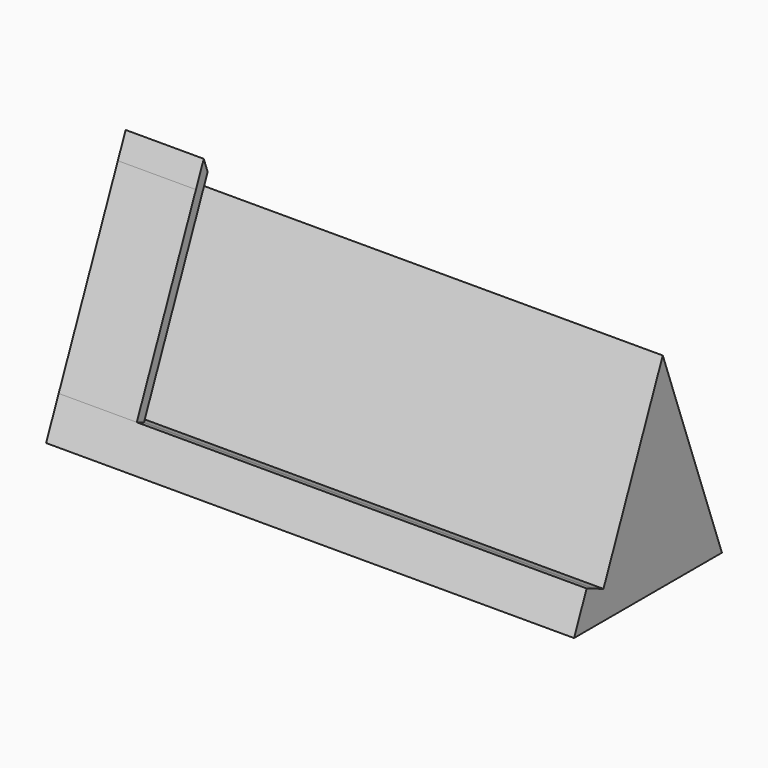
from build123d import *

# Parameters (mm, degrees)
F1_DEPTH = 57.6
F2_DEPTH = 5
F3_START = -5
F3_DEPTH = 5


# Not quite as in the source:
# - a feature names something its author has since deleted; it is built from what else it names


with BuildPart() as f1:
    # F0 (on Right) → F1 (new body)
    with BuildSketch(Plane.YZ):
        Polygon((1.5365748771, 3.633035603), (0, 0), (20.4984284937, 0), (11.0311029763, 26.0816380962), align=None)
        Polygon((0, 4.2829225325), (0, 0), (1.5365748771, 3.633035603), align=None)
        Polygon((-1.811441418, 0), (0, 0), (0, 4.2829225325), align=None)
        Polygon((-1.811441418, 0), (0, 4.2829225325), (-1.1518723498, 4.7701013845), (-3.1693637124, 0), align=None)
    extrude(amount=F1_DEPTH)

    # F0 (on Right) → F2 (join)
    with BuildSketch(Plane.YZ):
        Polygon((-1.1518723498, 4.7701013845), (0, 4.2829225325), (9.4668246651, 26.666023784), (10.1944775948, 28.3864664644), (9.5673128152, 30.1142495409), (8.3149523153, 27.153202636), align=None)
        Polygon((1.5365748771, 3.633035603), (0, 0), (20.4984284937, 0), (11.0311029763, 26.0816380962), align=None)
        Polygon((-1.811441418, 0), (0, 0), (0, 4.2829225325), align=None)
        Polygon((-1.811441418, 0), (0, 4.2829225325), (-1.1518723498, 4.7701013845), (-3.1693637124, 0), align=None)
        Polygon((0, 4.2829225325), (0, 0), (1.5365748771, 3.633035603), align=None)
    extrude(amount=-F2_DEPTH)

    # F0 (on Right) → F3 (join)
    with BuildSketch(Plane.YZ.offset(F3_START)):
        Polygon((-1.1518723498, 4.7701013845), (0, 4.2829225325), (9.4668246651, 26.666023784), (10.1944775948, 28.3864664644), (9.5673128152, 30.1142495409), (8.3149523153, 27.153202636), align=None)
        Polygon((0, 4.2829225325), (1.5365748771, 3.633035603), (11.0311029763, 26.0816380962), (10.1944775948, 28.3864664644), (9.4668246651, 26.666023784), align=None)
        Polygon((1.5365748771, 3.633035603), (0, 0), (20.4984284937, 0), (11.0311029763, 26.0816380962), align=None)
        Polygon((0, 4.2829225325), (0, 0), (1.5365748771, 3.633035603), align=None)
        Polygon((-1.811441418, 0), (0, 0), (0, 4.2829225325), align=None)
        Polygon((-1.811441418, 0), (0, 4.2829225325), (-1.1518723498, 4.7701013845), (-3.1693637124, 0), align=None)
    extrude(amount=-F3_DEPTH)


solid = f1.part
